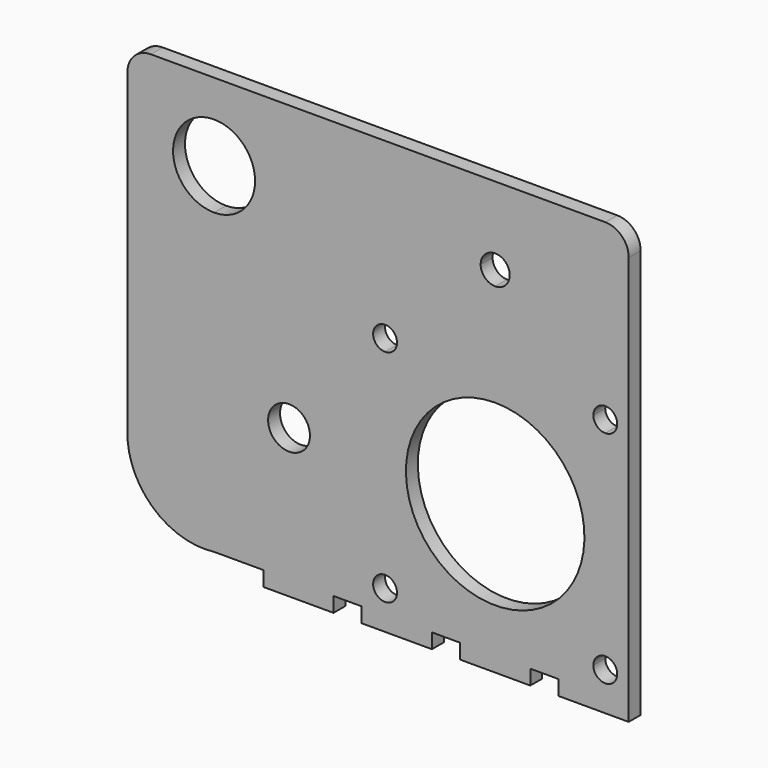
from build123d import *

# Parameters (mm, degrees)
F0_W     = 15
F0_H     = 3.175
F0_W_2   = 7.5
F0_R     = 4.4670073426
F1_DEPTH = 3.175


# Not quite as in the source:
# - a feature names something its author has since deleted; it is built from what else it names


with BuildPart() as f1:
    # F0 (on Front) → F1 (new body)
    with BuildSketch(Plane.XZ):
        with BuildLine():
            Line((0, 19.05), (0, 23.5))
            Line((0, 23.5), (-20.95, 23.5))
            ThreePointArc((-20.95, 23.5), (-21.696877708, 21.696877708), (-23.5, 20.95))
            Line((-23.5, 20.95), (-23.5, 0))
            Line((-23.5, 0), (-19.05, 0))
            ThreePointArc((-19.05, 0), (-13.4703841816, 13.4703841816), (0, 19.05))
        make_face()
        with BuildLine():
            Line((20.95, 23.5), (0, 23.5))
            Line((0, 23.5), (0, 19.05))
            ThreePointArc((0, 19.05), (13.4703841816, 13.4703841816), (19.05, 0))
            ThreePointArc((19.05, 0), (0, -19.05), (-19.05, 0))
            Line((-19.05, 0), (-23.5, 0))
            Line((-23.5, 0), (-23.5, -20.95))
            ThreePointArc((-23.5, -20.95), (-21.696877708, -21.696877708), (-20.95, -23.5))
            Line((-20.95, -23.5), (20.95, -23.5))
            ThreePointArc((20.95, -23.5), (21.696877708, -21.696877708), (23.5, -20.95))
            Line((23.5, -20.95), (23.5, 20.95))
            ThreePointArc((23.5, 20.95), (21.696877708, 21.696877708), (20.95, 23.5))
        make_face()
        with Locations((21, -30.0875)):
            Rectangle(F0_W, F0_H)
        with Locations((3.75, -30.0875)):
            Rectangle(F0_W_2, F0_H)
        with Locations((-3.75, -30.0875)):
            Rectangle(F0_W_2, F0_H)
        with Locations((-21, -30.0875)):
            Rectangle(F0_W, F0_H)
        with BuildLine():
            Line((0, 28.5), (-28.5, 28.5))
            Line((-28.5, 28.5), (-28.5, 0))
            Line((-28.5, 0), (-23.5, 0))
            Line((-23.5, 0), (-23.5, 20.95))
            ThreePointArc((-23.5, 20.95), (-25.303122292, 25.303122292), (-20.95, 23.5))
            Line((-20.95, 23.5), (0, 23.5))
            Line((0, 23.5), (0, 28.5))
        make_face()
        with BuildLine():
            Line((23.5, 28.5), (0, 28.5))
            Line((0, 28.5), (0, 23.5))
            Line((0, 23.5), (20.95, 23.5))
            ThreePointArc((20.95, 23.5), (23.5, 26.05), (26.05, 23.5))
            ThreePointArc((26.05, 23.5), (25.303122292, 21.696877708), (23.5, 20.95))
            Line((23.5, 20.95), (23.5, -20.95))
            ThreePointArc((23.5, -20.95), (25.303122292, -21.696877708), (26.05, -23.5))
            ThreePointArc((26.05, -23.5), (23.5, -26.05), (20.95, -23.5))
            Line((20.95, -23.5), (-20.95, -23.5))
            ThreePointArc((-20.95, -23.5), (-25.303122292, -25.303122292), (-23.5, -20.95))
            Line((-23.5, -20.95), (-23.5, 0))
            Line((-23.5, 0), (-28.5, 0))
            Line((-28.5, 0), (-28.5, -28.5))
            Line((-28.5, -28.5), (-13.5, -28.5))
            Line((-13.5, -28.5), (-7.5, -28.5))
            Line((-7.5, -28.5), (0, -28.5))
            Line((0, -28.5), (7.5, -28.5))
            Line((7.5, -28.5), (13.5, -28.5))
            Line((13.5, -28.5), (28.5, -28.5))
            Line((28.5, -28.5), (28.5, 23.5))
            Line((28.5, 23.5), (28.5, 28.5))
            Line((28.5, 28.5), (23.5, 28.5))
        make_face()
        with BuildLine():
            Line((-51.25, 44), (-28.5, 44))
            Line((-28.5, 44), (-28.5, 60.5991594493))
            Line((-28.5, 60.5991594493), (-73.5, 60.5991594493))
            ThreePointArc((-73.5, 60.5991594493), (-77.0355339059, 59.1346933553), (-78.5, 55.5991594493))
            Line((-78.5, 55.5991594493), (-78.5, -11.5))
            ThreePointArc((-78.5, -11.5), (-73.1911039749, -24.2888484433), (-60, -28.5))
            Line((-60, -28.5), (-60, 35.25))
            ThreePointArc((-60, 35.25), (-66.1871843354, 50.1871843354), (-51.25, 44))
        make_face()
        with BuildLine():
            Line((-28.5, 0), (-28.5, 28.5))
            Line((-28.5, 28.5), (-28.5, 44))
            Line((-28.5, 44), (-51.25, 44))
            ThreePointArc((-51.25, 44), (-53.8128156646, 37.8128156646), (-60, 35.25))
            Line((-60, 35.25), (-60, -28.5))
            Line((-60, -28.5), (-49.5, -28.5))
            Line((-49.5, -28.5), (-34.5, -28.5))
            Line((-34.5, -28.5), (-28.5, -28.5))
            Line((-28.5, -28.5), (-28.5, 0))
        make_face()
        with Locations((-44, 0)):
            Circle(F0_R, mode=Mode.SUBTRACT)
        with Locations((-42, -30.0875)):
            Rectangle(F0_W, F0_H)
        with BuildLine():
            Line((-28.5, 44), (-28.5, 28.5))
            Line((-28.5, 28.5), (0, 28.5))
            Line((0, 28.5), (0, 40.9))
            ThreePointArc((0, 40.9), (-2.1920310217, 41.8079689783), (-3.1, 44))
            Line((-3.1, 44), (-28.5, 44))
        make_face()
        with BuildLine():
            Line((0, 40.9), (0, 28.5))
            Line((0, 28.5), (23.5, 28.5))
            Line((23.5, 28.5), (28.5, 28.5))
            Line((28.5, 28.5), (28.5, 55.5991594493))
            ThreePointArc((28.5, 55.5991594493), (27.0355339059, 59.1346933553), (23.5, 60.5991594493))
            Line((23.5, 60.5991594493), (-28.5, 60.5991594493))
            Line((-28.5, 60.5991594493), (-28.5, 44))
            Line((-28.5, 44), (-3.1, 44))
            ThreePointArc((-3.1, 44), (0, 47.1), (3.1, 44))
            ThreePointArc((3.1, 44), (2.1920310217, 41.8079689783), (0, 40.9))
        make_face()
    extrude(amount=F1_DEPTH)


solid = f1.part
